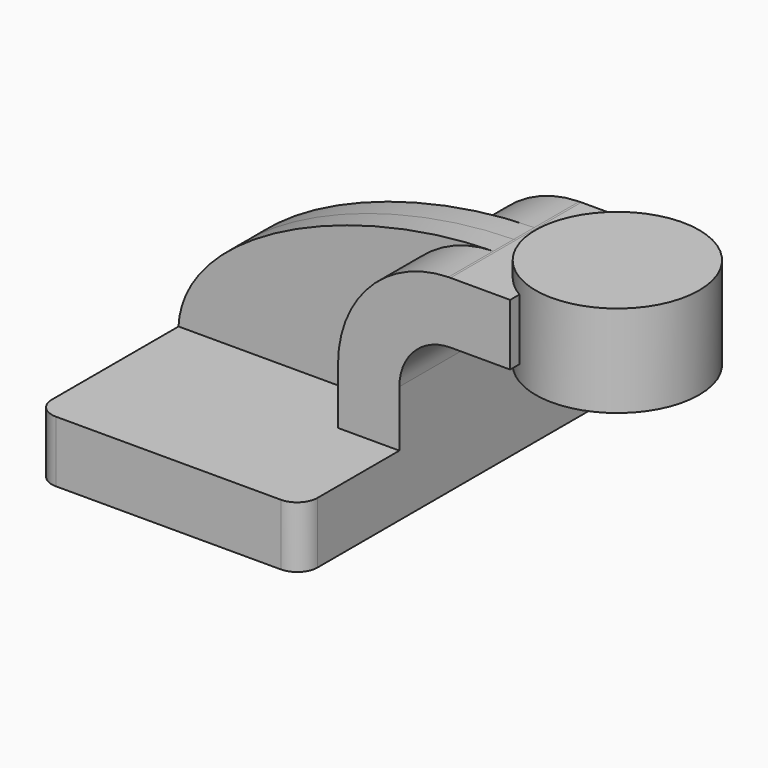
from build123d import *

# Parameters (mm, degrees)
F1_DEPTH = 63.5
F2_R     = 6.35
F0_W     = 25.4
F0_H     = 28.575
F4_DEPTH = 7.9375
F0_W_2   = 12.4209585713
F0_H_2   = 19.05
F5_DEPTH = 25.4


with BuildPart() as f1:
    # F0 (on Front) → F1 (new body, symmetric)
    with BuildSketch(Plane.XZ):
        Polygon((22.225, 9.525), (-41.275, 9.525), (-41.275, -9.525), (41.275, -9.525), (41.275, 9.525), align=None)
    extrude(amount=F1_DEPTH, both=True)

    # F2
    f2_edges = [f1.edges().sort_by_distance(p)[0] for p in [
        (41.275, -63.5, 0),
        (-41.275, -63.5, 0),
        (-41.275, 63.5, 0),
        (41.275, 63.5, 0),
    ]]
    fillet(f2_edges, radius=F2_R)

    # F0 (on Front) → F4 (join, symmetric)
    with BuildSketch(Plane.XZ):
        with BuildLine():
            add(Edge.make_bspline(
                [(56.5045744803, 61.9192356525), (12.1359940595, 61.3987338725), (-39.902945727, 38.0672359689), (-41.275, 9.525)],
                knots=[0.538528036, 0.538528036, 0.538528036, 0.538528036, 111.5045361635, 111.5045361635, 111.5045361635, 111.5045361635], degree=3))
            Line((-41.275, 9.525), (22.225, 9.525))
            Line((22.225, 9.525), (22.225, 27.0002))
            ThreePointArc((22.225, 27.0002), (32.2271479233, 51.4666478289), (56.5045744803, 61.9192356525))
        make_face()
    extrude(amount=F4_DEPTH, both=True)

    # F0 (on Front) → F5 (join, symmetric)
    with BuildSketch(Plane.XZ):
        with BuildLine():
            Line((22.225, 27.0002), (22.225, 9.525))
            Line((22.225, 9.525), (41.275, 9.525))
            Line((41.275, 9.525), (41.275, 27.0002))
            ThreePointArc((41.275, 27.0002), (45.9246798487, 38.2255201513), (57.15, 42.8752))
            Line((57.15, 42.8752), (63.257267818, 42.8752))
            Line((63.257267818, 42.8752), (63.257267818, 61.9252))
            Line((63.257267818, 61.9252), (57.15, 61.9252))
            add(Edge.make_bspline(
                [(57.15, 61.9252), (56.9350432615, 61.9237504809), (56.7198991989, 61.9217616945), (56.5045744803, 61.9192356525)],
                knots=[0, 0, 0, 0, 0.538528036, 0.538528036, 0.538528036, 0.538528036], degree=3))
            ThreePointArc((56.5045744803, 61.9192356525), (32.2271479233, 51.4666478289), (22.225, 27.0002))
        make_face()
        with Locations((69.4677471036, 52.4002)):
            Rectangle(F0_W_2, F0_H_2)
    extrude(amount=F5_DEPTH, both=True)


with BuildPart() as f3:
    # F0 (on Front) → F3 (revolve)
    with BuildSketch(Plane.XZ):
        with Locations((101.357267818, 52.3875)):
            Rectangle(F0_W, F0_H)
    revolve(axis=Axis((88.657267818, 0, 52.3875), (0, 0, 1)))


solid = Compound([f1.part, f3.part])
